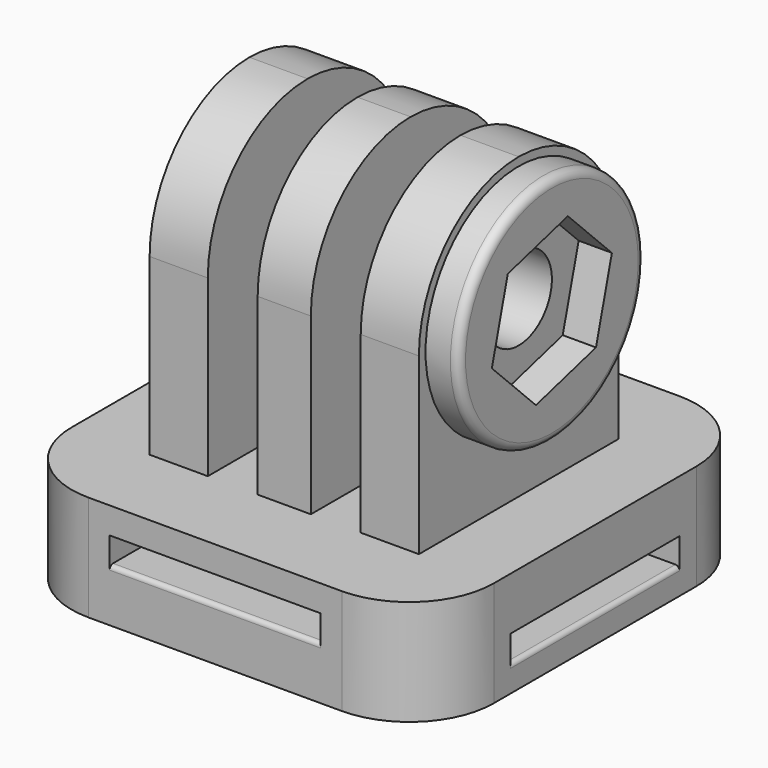
from build123d import *

# Parameters (mm, degrees)
F0_W      = 25.4
F0_H      = 25.4
F1_DEPTH  = 6.35
F2_W      = 12.7
F2_H      = 1.5875
F3_DEPTH  = 25.401
F4_W      = 12.7
F4_H      = 1.5875
F5_DEPTH  = 25.401
F6_W      = 3.5
F6_H      = 15
F6_W_2    = 3.2
F7_DEPTH  = 18
F8_R      = 7.49999
F9_R      = 5.08
F10_R     = 7
F11_DEPTH = 2
F12_D     = 5
F13_R     = 0.508
F14_R     = 0.254


# Not quite as in the source:
# - a fillet or chamfer is up to 0.001 mm smaller than in the source, because OpenCascade refuses the exact size


with BuildPart() as f1:
    # F0 (on Top) → F1 (new body)
    with BuildSketch(Plane.XY):
        Rectangle(F0_W, F0_H)
    extrude(amount=F1_DEPTH)

    # F2 (on face) → F3 (cut, through all)
    with BuildSketch(Plane.YZ.offset(12.7)):
        with Locations((0, 2.38125)):
            Rectangle(F2_W, F2_H)
    extrude(amount=-F3_DEPTH, mode=Mode.SUBTRACT)

    # F4 (on face) → F5 (cut, through all)
    with BuildSketch(Plane.XZ.offset(12.7)):
        with Locations((0, 3.96875)):
            Rectangle(F4_W, F4_H)
    extrude(amount=-F5_DEPTH, mode=Mode.SUBTRACT)

    # F6 (on face) → F7 (join)
    with BuildSketch(Plane.XY.offset(6.35)):
        with Locations((-6.35, 0)):
            Rectangle(F6_W, F6_H)
        Rectangle(F6_W_2, F6_H)
        with Locations((6.35, 0)):
            Rectangle(F6_W, F6_H)
    extrude(amount=F7_DEPTH)

    # F8 (radius 7.5 in the source; OpenCascade refuses exactly that, so slightly less here)
    f8_edges = [f1.edges().sort_by_distance(p)[0] for p in [
        (6.35, -7.5, 24.35),
        (0, -7.5, 24.35),
        (-6.35, -7.5, 24.35),
        (-6.35, 7.5, 24.35),
        (6.35, 7.5, 24.35),
        (0, 7.5, 24.35),
    ]]
    fillet(f8_edges, radius=F8_R)

    # F9
    f9_edges = [f1.edges().sort_by_distance(p)[0] for p in [
        (12.7, 12.7, 3.175),
        (12.7, -12.7, 3.175),
        (-12.7, 12.7, 3.175),
        (-12.7, -12.7, 3.175),
    ]]
    fillet(f9_edges, radius=F9_R)

    # F10 (on face) → F11 (join)
    with BuildSketch(Plane.YZ.offset(8.1)):
        with Locations((0, 16.85)):
            Circle(F10_R)
        Polygon((-4.5135996016, 15.6263094195), (-3.3165469299, 20.1470466272), (1.1970526717, 21.3707372077), (4.5135996016, 18.0736905805), (3.3165469299, 13.5529533728), (-1.1970526717, 12.3292627923), align=None, mode=Mode.SUBTRACT)
    extrude(amount=F11_DEPTH)

    # F12 (through all)
    with Locations(Plane.YZ.offset(8.1)):
        with Locations((0, 16.85)):
            Hole(F12_D / 2)

    # F13
    f13_edges = [f1.edges().sort_by_distance(p)[0] for p in [
        (10.1, -7, 16.85),
    ]]
    fillet(f13_edges, radius=F13_R)

    # F14
    f14_edges = [f1.edges().sort_by_distance(p)[0] for p in [
        (-12.7, 0, 1.5875),
        (0, -12.7, 3.175),
        (12.7, 0, 1.5875),
        (0, 12.7, 3.175),
    ]]
    fillet(f14_edges, radius=F14_R)


solid = f1.part
